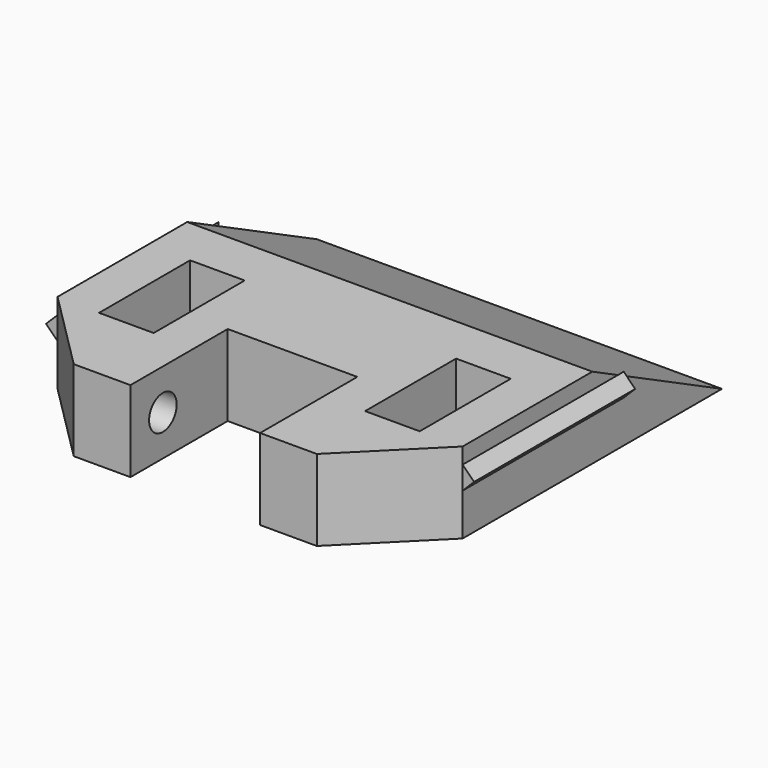
from build123d import *

# Parameters (mm, degrees)
F1_DEPTH  = 50.8
F3_DEPTH  = 254.001
F4_W      = 81.28
F4_H      = 76.2
F5_DEPTH  = 50.801
F7_DEPTH  = 177.038
F8_W      = 14.2059672672
F8_H      = 54.5313454777
F8_W_2    = 25.0834482712
F8_H_2    = 56.1428241044
F9_DEPTH  = 50.801
F10_W     = 34.2439590022
F10_H     = 71.3080037385
F11_DEPTH = 50.801
F12_R     = 10.795
F13_DEPTH = 25.4
F14_R     = 10.795
F15_DEPTH = 25.4


# Not quite as in the source:
# - a feature names something its author has since deleted; it is built from what else it names


with BuildPart() as f1:
    # F0 (on Top) → F1 (new body)
    with BuildSketch(Plane.XY):
        Polygon((208.3008480269, 184.2279704243), (-45.6991519731, 184.2279704243), (-45.6991519731, -18.9720295757), (5.1008480269, -69.7720295757), (157.5008480269, -69.7720295757), (208.3008480269, -18.9720295757), align=None)
    extrude(amount=F1_DEPTH)

    # F2 (on face) → F3 (cut, through all)
    with BuildSketch(Plane.YZ.offset(208.3008480269)):
        Polygon((82.6279704243, 50.8), (184.2279704243, 0), (184.2279704243, 50.8), align=None)
    extrude(amount=-F3_DEPTH, mode=Mode.SUBTRACT)

    # F4 (on face) → F5 (cut, through all)
    with BuildSketch(Plane.XY.offset(50.8)):
        with Locations((81.3008480269, -31.6720295757)):
            Rectangle(F4_W, F4_H)
    extrude(amount=-F5_DEPTH, mode=Mode.SUBTRACT)

    # F6 (on face) → F7 (join)
    with BuildSketch(Plane.XZ.offset(69.7720295757)):
        Polygon((-52.88335687, 33.5843649413), (-45.6991519731, 26.4001600444), (-45.6991519731, 40.7685698381), align=None)
        Polygon((208.3008480269, 26.4001600444), (215.4850529237, 33.5843649413), (208.3008480269, 40.7685698381), align=None)
    extrude(amount=-F7_DEPTH)

    # F8 (on face) → F9 (cut, through all)
    with BuildSketch(Plane.XY.offset(50.8)):
        with Locations((-52.8021356067, -46.2377023146)):
            Rectangle(F8_W, F8_H)
        with Locations((220.8425721625, -47.0434416279)):
            Rectangle(F8_W_2, F8_H_2)
    extrude(amount=-F9_DEPTH, mode=Mode.SUBTRACT)

    # F10 (on face) → F11 (cut, through all)
    with BuildSketch(Plane.XY.offset(50.8)):
        with Locations((-2.0932615735, 16.1352222785)):
            Rectangle(F10_W, F10_H)
        with Locations((164.6949576272, 16.1352222785)):
            Rectangle(F10_W, F10_H)
    extrude(amount=-F11_DEPTH, mode=Mode.SUBTRACT)

    # F12 (on face) → F13 (cut)
    with BuildSketch(Plane.YZ.offset(40.6608480269)):
        with Locations((-44.3720295757, 25.4)):
            Circle(F12_R)
    extrude(amount=-F13_DEPTH, mode=Mode.SUBTRACT)

    # F14 (on face) → F15 (cut)
    with BuildSketch(Plane(origin=(121.9408480269, 0, 0), x_dir=(0, -1, 0), z_dir=(-1, 0, 0))):
        with Locations((44.3720295757, 25.4)):
            Circle(F14_R)
    extrude(amount=-F15_DEPTH, mode=Mode.SUBTRACT)


solid = f1.part
